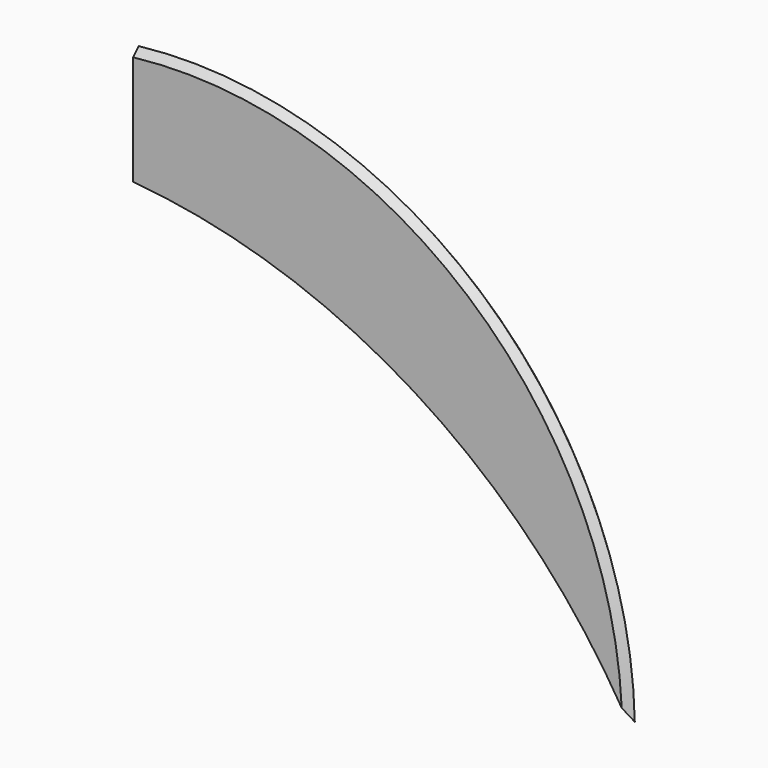
from build123d import *

# Parameters (mm, degrees)
F1_DEPTH = 3
F2_SIZE  = 1.49999


# Not quite as in the source:
# - a fillet or chamfer is up to 0.001 mm smaller than in the source, because OpenCascade refuses the exact size


with BuildPart() as f1:
    # F0 (on Front) → F1 (new body)
    with BuildSketch(Plane.XZ):
        with BuildLine():
            ThreePointArc((0, 0), (61.4781903769, -20.8298692006), (106.2082496532, -67.8689289283))
            ThreePointArc((106.2082496532, -67.8689289283), (73.6372514953, 2.0479582207), (0, 25))
            Line((0, 25), (0, 0))
        make_face()
    extrude(amount=F1_DEPTH)

    # F2 (size 1.5 in the source; OpenCascade refuses exactly that, so slightly less here)
    f2_edges = [f1.edges().sort_by_distance(p)[0] for p in [
        (73.637251, -3, 2.047958),
        (73.637251, 0, 2.047958),
    ]]
    chamfer(f2_edges, length=F2_SIZE)


solid = f1.part
